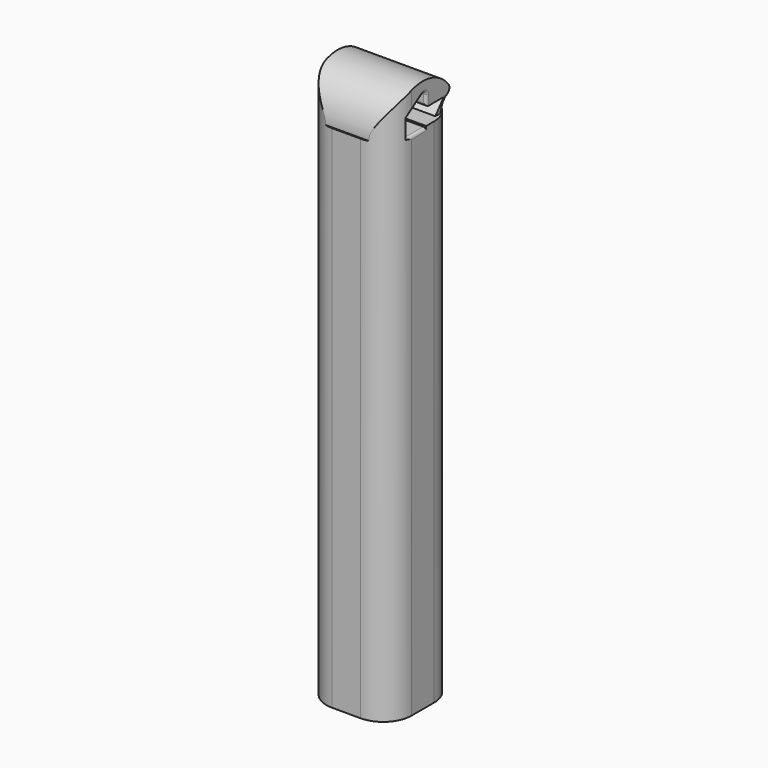
from build123d import *

# Parameters (mm, degrees)
F0_W         = 15
F0_H         = 90
F1_DEPTH     = 15
F3_DEPTH     = 7.5
F4_DEPTH     = 7.5
F5_F1_R      = 0.5
F5_F2_R      = 0.5
F6_R         = 0.5
F7_T1_DEPTH  = 24.4510456068
F8_T1_DEPTH  = 115
F8_T6_DEPTH  = 115
F8_T11_DEPTH = 115


# Not quite as in the source:
# - a fillet or chamfer that OpenCascade refuses, or shapes differently, is made with other operations: its cross-section is extruded or revolved along the edge and cut away or added


with BuildPart() as f1:
    # F0 (on Front) → F1 (new body)
    with BuildSketch(Plane.XZ):
        Rectangle(F0_W, F0_H)
    extrude(amount=F1_DEPTH)

    # F2 (on Right) → F3 (join, symmetric)
    with BuildSketch(Plane.YZ):
        with BuildLine():
            Line((-2.532008104, 48.1942993341), (-0.9043752619, 48.1942993341))
            ThreePointArc((-0.9043752619, 48.1942993341), (-14.6602935003, 43.7750522985), (-0.289426955, 45.269450398))
            Line((-0.289426955, 45.269450398), (-6.7935246953, 45.269450398))
            Line((-6.7935246953, 45.269450398), (-6.7935246953, 43.9416393638))
            Line((-6.7935246953, 43.9416393638), (-10.9625607729, 43.9416393638))
            Line((-10.9625607729, 43.9416393638), (-10.9625607729, 48.1942993341))
            Line((-10.9625607729, 48.1942993341), (-6.7935246953, 50.9531982243))
            Line((-6.7935246953, 50.9531982243), (-6.7935246953, 48.1942993341))
            Line((-6.7935246953, 48.1942993341), (-2.9029950965, 48.1942993341))
            Line((-2.9029950965, 48.1942993341), (-2.532008104, 48.1942993341))
        make_face()
    extrude(amount=F3_DEPTH, both=True)

    # F2 (on Right) → F4 (join, symmetric)
    with BuildSketch(Plane.YZ):
        Polygon((-3.1812353409, 47.4117453826), (-2.9029950965, 48.1942993341), (-4.7579342499, 45.9584258497), (-3.6979690194, 45.9584258497), align=None)
        Polygon((-3.1812353409, 47.4117453826), (-2.532008104, 48.1942993341), (-2.9029950965, 48.1942993341), align=None)
    extrude(amount=F4_DEPTH, both=True)

    # F5: fillet of radius 0.5 on 7 edges, made by hand

    # F5_f1
    f5_f1_edges = [f1.edges().sort_by_distance(p)[0] for p in [
        (0, -6.7935246953, 50.9531982243),
    ]]
    fillet(f5_f1_edges, radius=F5_F1_R)

    # F5_f2
    f5_f2_edges = [f1.edges().sort_by_distance(p)[0] for p in [
        (7.5, -9.2660086927, 49.3170086521),
        (7.5, -10.9625607729, 46.597149667),
        (7.5, -8.8780427341, 45),
        (-7.5, -6.7935246953, 49.1085250933),
        (0, -6.7935246953, 48.1942993341),
        (7.5, -6.7935246953, 49.1085250933),
        (7.5, -7.0568455439, 50.4631858413),
        (-7.5, -7.0568455439, 50.4631858413),
    ]]
    fillet(f5_f2_edges, radius=F5_F2_R)

    # F6
    f6_edges = [f1.edges().sort_by_distance(p)[0] for p in [
        (-7.5, -8.878043, 45),
        (-7.5, -10.962561, 46.59715),
    ]]
    fillet(f6_edges, radius=F6_R)

    # F7: fillet of radius 1 on 1 edges, made by hand

    # F7_s2 → F7_t1 (cut)
    with BuildSketch(Plane.YZ.offset(-12.2255228034)):
        with BuildLine():
            ThreePointArc((-1.8842228199, 49.8107118079), (-1.7364138721, 48.8134688286), (-2.532008104, 48.1942993341))
            Line((-2.532008104, 48.1942993341), (-0.9043752619, 48.1942993341))
            ThreePointArc((-0.9043752619, 48.1942993341), (-1.3414912221, 49.0345169623), (-1.8842228199, 49.8107118079))
        make_face()
    extrude(amount=F7_T1_DEPTH, mode=Mode.SUBTRACT)

    # F8: fillet of radius 5 on 4 edges, made by hand

    # F8_s2 → F8_t1 (cut)
    with BuildSketch(Plane.XY.offset(-57.5)):
        with BuildLine():
            ThreePointArc((-7.5, -10), (-6.0355339059, -13.5355339059), (-2.5, -15))
            Line((-2.5, -15), (-7.5, -15))
            Line((-7.5, -15), (-7.5, -10))
        make_face()
        with BuildLine():
            ThreePointArc((7.5, -10), (6.0355339059, -13.5355339059), (2.5, -15))
            Line((2.5, -15), (7.5, -15))
            Line((7.5, -15), (7.5, -10))
        make_face()
    extrude(amount=F8_T1_DEPTH, mode=Mode.SUBTRACT)


with BuildPart() as f8_tool4:
    # F8_s5 → F8_t6 (new body)
    with BuildSketch(Plane.XY.offset(57.5)):
        with BuildLine():
            ThreePointArc((-7.5, -5), (-6.0355339059, -1.4644660941), (-2.5, 0))
            Line((-2.5, 0), (-7.5, 0))
            Line((-7.5, 0), (-7.5, -5))
        make_face()
    extrude(amount=-F8_T6_DEPTH)

    split(bisect_by=Plane.XY.offset(45.269450398), keep=Keep.BOTTOM)


with BuildPart() as f1_1:
    add(f1.part)

    # F8_t3: cut F8_tool4
    add(f8_tool4.part, mode=Mode.SUBTRACT)


with BuildPart() as f8_tool9:
    # F8_s10 → F8_t11 (new body)
    with BuildSketch(Plane.XY.offset(-57.5)):
        with BuildLine():
            ThreePointArc((7.5, -5), (6.0355339059, -1.4644660941), (2.5, 0))
            Line((2.5, 0), (7.5, 0))
            Line((7.5, 0), (7.5, -5))
        make_face()
    extrude(amount=F8_T11_DEPTH)

    split(bisect_by=Plane.XY.offset(45.269450398), keep=Keep.BOTTOM)


with BuildPart() as f1_2:
    add(f1_1.part)

    # F8_t8: cut F8_tool9
    add(f8_tool9.part, mode=Mode.SUBTRACT)


solid = f1_2.part
